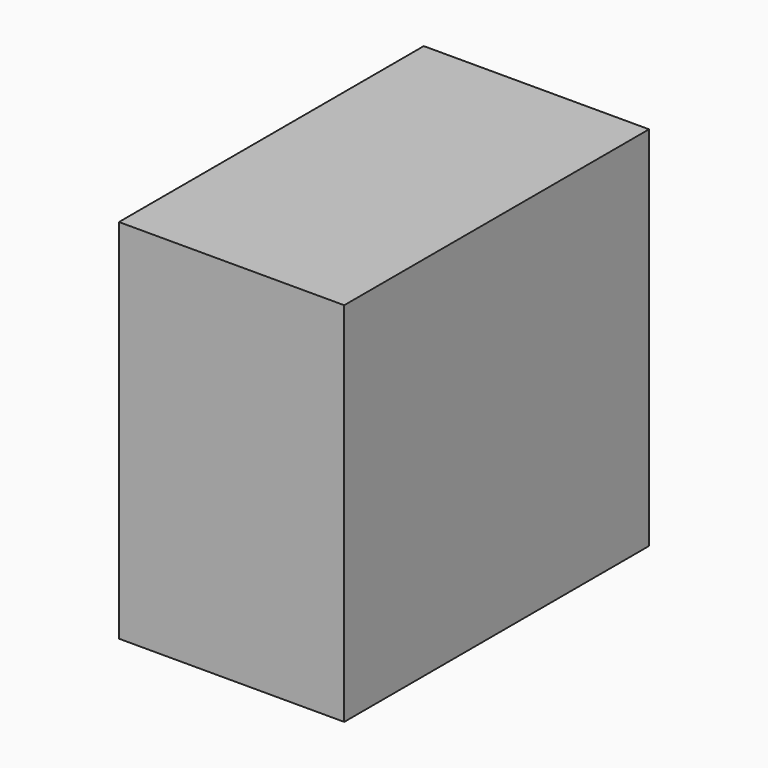
from build123d import *

# Parameters (mm, degrees)
F1_DEPTH = 12.7


# Not quite as in the source:
# - the program builds the solid bodies; features that only make, move or delete a surface that nothing else refers to are left out


with BuildPart() as f1:
    # F0 (on Right) → F1 (new body, symmetric)
    with BuildSketch(Plane.YZ):
        with BuildLine():
            Line((-42.9621189833, 0), (0, 0))
            Line((0, 0), (0, 15.7109107822))
            Line((0, 15.7109107822), (-7.3093525134, 15.7109107822))
            ThreePointArc((-7.3093525134, 15.7109107822), (-19.2494977024, 19.8276732117), (-7.3093525134, 23.9444356412))
            Line((-7.3093525134, 23.9444356412), (0, 23.9444356412))
            Line((0, 23.9444356412), (0, 41.3635261357))
            Line((0, 41.3635261357), (-42.9621189833, 41.3635261357))
            Line((-42.9621189833, 41.3635261357), (-42.9621189833, 0))
        make_face()
        with BuildLine():
            Line((-7.3093525134, 15.7109107822), (0, 15.7109107822))
            Line((0, 15.7109107822), (0, 23.9444356412))
            Line((0, 23.9444356412), (-7.3093525134, 23.9444356412))
            ThreePointArc((-7.3093525134, 23.9444356412), (-19.2494977024, 19.8276732117), (-7.3093525134, 15.7109107822))
        make_face()
    extrude(amount=F1_DEPTH, both=True)


solid = f1.part
